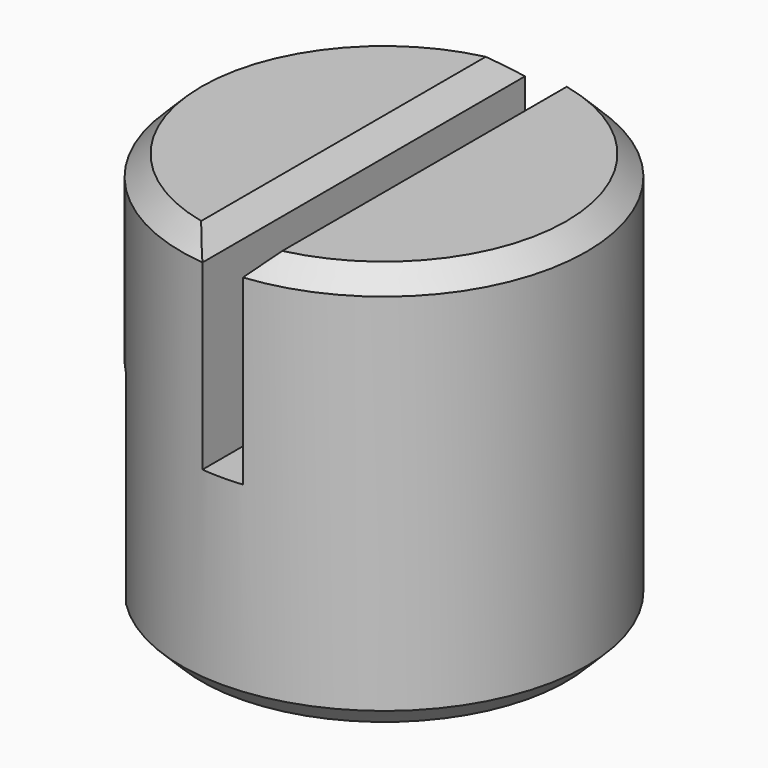
from build123d import *
from build123d import SkipClean  # not in build123d's __all__

# Parameters (mm, degrees)
F1_DEPTH     = 5
F2_DEPTH     = 5
F3_T3_DEPTH  = 12.521557359
F3_T6_ANGLE  = 198.0325102457
F3_T9_ANGLE  = 198.0325102457
F3_T12_DEPTH = 12.521557359
F3_T15_ANGLE = 209.516708524
F3_T18_DEPTH = 12.571682988
F3_T21_ANGLE = 144.0077008654
F3_T24_ANGLE = 53.9966137912
F3_T27_DEPTH = 7.0466201735
F3_T31_DEPTH = 8.0466201735


# Not quite as in the source:
# - a fillet or chamfer that OpenCascade refuses, or shapes differently, is made with other operations: its cross-section is extruded or revolved along the edge and cut away or added


with BuildPart() as f1:
    # F0 (on Top) → F1 (new body)
    with BuildSketch(Plane.XY):
        with BuildLine():
            ThreePointArc((-3.5355339059, -3.5355339059), (-2.1422777427, -4.5178143026), (-0.5, -4.9749371855))
            Line((-0.5, -4.9749371855), (-0.5, -0.5))
            Line((-0.5, -0.5), (-3.5355339059, -3.5355339059))
        make_face()
        with BuildLine():
            ThreePointArc((-0.5, -4.9749371855), (-0.2503138753, -4.9937303656), (0, -5))
            Line((0, -5), (0, 0))
            Line((0, 0), (-0.5, -0.5))
            Line((-0.5, -0.5), (-0.5, -4.9749371855))
        make_face()
        with BuildLine():
            ThreePointArc((0, -5), (0.2503138753, -4.9937303656), (0.5, -4.9749371855))
            Line((0.5, -4.9749371855), (0.5, 0.5))
            Line((0.5, 0.5), (0, 0))
            Line((0, 0), (0, -5))
        make_face()
        with BuildLine():
            ThreePointArc((0.5, -4.9749371855), (3.7080992435, -3.3541019662), (5, 0))
            ThreePointArc((5, 0), (4.6193976626, 1.9134171618), (3.5355339059, 3.5355339059))
            Line((3.5355339059, 3.5355339059), (0.5, 0.5))
            Line((0.5, 0.5), (0.5, -4.9749371855))
        make_face()
    extrude(amount=-F1_DEPTH)

    # F0 (on Top) → F2 (join)
    with BuildSketch(Plane.XY):
        with BuildLine():
            Line((-0.5, -0.5), (-0.5, 4.9749371855))
            ThreePointArc((-0.5, 4.9749371855), (-4.7093962486, 1.6797580105), (-3.5355339059, -3.5355339059))
            Line((-3.5355339059, -3.5355339059), (-0.5, -0.5))
        make_face()
        with BuildLine():
            Line((0.5, 0.5), (3.5355339059, 3.5355339059))
            ThreePointArc((3.5355339059, 3.5355339059), (2.1422777427, 4.5178143026), (0.5, 4.9749371855))
            Line((0.5, 4.9749371855), (0.5, 0.5))
        make_face()
        with BuildLine():
            ThreePointArc((0.5, -4.9749371855), (3.7080992435, -3.3541019662), (5, 0))
            ThreePointArc((5, 0), (4.6193976626, 1.9134171618), (3.5355339059, 3.5355339059))
            Line((3.5355339059, 3.5355339059), (0.5, 0.5))
            Line((0.5, 0.5), (0.5, -4.9749371855))
        make_face()
        with BuildLine():
            ThreePointArc((-3.5355339059, -3.5355339059), (-2.1422777427, -4.5178143026), (-0.5, -4.9749371855))
            Line((-0.5, -4.9749371855), (-0.5, -0.5))
            Line((-0.5, -0.5), (-3.5355339059, -3.5355339059))
        make_face()
    with SkipClean():  # cleaning this boolean's faces spoils the solid; the shape is the same uncleaned
        extrude(amount=F2_DEPTH)

    # F3: chamfer of 0.5 on 12 edges, made by hand


with BuildPart() as f3_tool1:
    # F3_s2 → F3_t3 (new body)
    with BuildSketch(Plane.XZ.offset(-6.2607786795)):
        Polygon((0.5, 4.5), (1, 5), (0.5, 5), align=None)
    extrude(amount=F3_T3_DEPTH)


with BuildPart() as f3_tool4:
    # F3_s5 → F3_t6 (revolve)
    with BuildSketch(Plane(origin=(0, 0, 0), x_dir=(0, 0, 1), z_dir=(-0.9876439195, 0.1567146713, 0))):
        Polygon((4.5, -5), (5, -4.5), (5, -5), align=None)
    revolve(axis=Axis((0, 0, 5), (0, 0, 1)), revolution_arc=F3_T6_ANGLE)


with BuildPart() as f3_tool7:
    # F3_s8 → F3_t9 (revolve)
    with BuildSketch(Plane(origin=(0, 0, 0), x_dir=(0, 0, 1), z_dir=(0.9876439195, -0.1567146713, 0))):
        Polygon((4.5, -5), (5, -4.5), (5, -5), align=None)
    revolve(axis=Axis((0, 0, 5), (0, 0, 1)), revolution_arc=F3_T9_ANGLE)


with BuildPart() as f3_tool10:
    # F3_s11 → F3_t12 (new body)
    with BuildSketch(Plane.XZ.offset(6.2607786795)):
        Polygon((-0.5, 4.5), (-1, 5), (-0.5, 5), align=None)
    extrude(amount=-F3_T12_DEPTH)


with BuildPart() as f3_tool13:
    # F3_s14 → F3_t15 (revolve)
    with BuildSketch(Plane(origin=(0, 0, 0), x_dir=(0, 0, 1), z_dir=(-0.5036480164, 0.863908951, 0))):
        Polygon((-4.5, -5), (-5, -4.5), (-5, -5), align=None)
    revolve(axis=Axis((0, 0, -5), (0, 0, 1)), revolution_arc=F3_T15_ANGLE)


with BuildPart() as f3_tool16:
    # F3_s17 → F3_t18 (new body)
    with BuildSketch(Plane(origin=(4.4447611459, 4.4447611459, 0), x_dir=(0, 0, 1), z_dir=(-0.7071067812, -0.7071067812, 0))):
        Polygon((-4.5, 0), (-5, -0.5), (-5, 0), align=None)
    extrude(amount=F3_T18_DEPTH)


with BuildPart() as f3_tool19:
    # F3_s20 → F3_t21 (revolve)
    with BuildSketch(Plane(origin=(0, 0, 0), x_dir=(0, 0, 1), z_dir=(0.987667306, -0.1565672143, 0))):
        Polygon((0.5, -5), (0, -4.5), (0, -5), align=None)
    revolve(axis=Axis((0, 0, 0), (0, 0, 1)), revolution_arc=F3_T21_ANGLE)


with BuildPart() as f3_tool22:
    # F3_s23 → F3_t24 (revolve)
    with BuildSketch(Plane(origin=(0, 0, 0), x_dir=(0, 0, 1), z_dir=(0.7071067812, -0.7071067812, 0))):
        Polygon((0.5, -5), (0, -4.5), (0, -5), align=None)
    revolve(axis=Axis((0, 0, 0), (0, 0, 1)), revolution_arc=F3_T24_ANGLE)


with BuildPart() as f3_tool25:
    # F3_s26 → F3_t27 (new body)
    with BuildSketch(Plane.XZ.offset(-6.2607786795)):
        Polygon((1, 0), (0.5, 0.5), (0.5, 0), align=None)
    extrude(amount=F3_T27_DEPTH)

    split(bisect_by=Plane(origin=(0, 0, 0), x_dir=(0, 0, 1), z_dir=(-0.7071067812, 0.7071067812, 0)), keep=Keep.TOP)


with BuildPart() as f3_tool29:
    # F3_s30 → F3_t31 (new body)
    with BuildSketch(Plane.XZ.offset(1.785841494)):
        Polygon((-1, 0), (-0.5, 0.5), (-0.5, 0), align=None)
    extrude(amount=-F3_T31_DEPTH)

    split(bisect_by=Plane(origin=(0, 0, 0), x_dir=(0, 0, 1), z_dir=(-0.7071067812, 0.7071067812, 0)), keep=Keep.TOP)


with BuildPart() as f1_1:
    add(f1.part, clean=False)

    # F3_t33: cut F3_tool1, F3_tool4, F3_tool7, F3_tool10, F3_tool13, F3_tool16, F3_tool19, F3_tool22, F3_tool25, F3_tool29
    add([f3_tool1.part, f3_tool4.part, f3_tool7.part, f3_tool10.part, f3_tool13.part, f3_tool16.part, f3_tool19.part, f3_tool22.part, f3_tool25.part, f3_tool29.part], mode=Mode.SUBTRACT)


solid = f1_1.part
